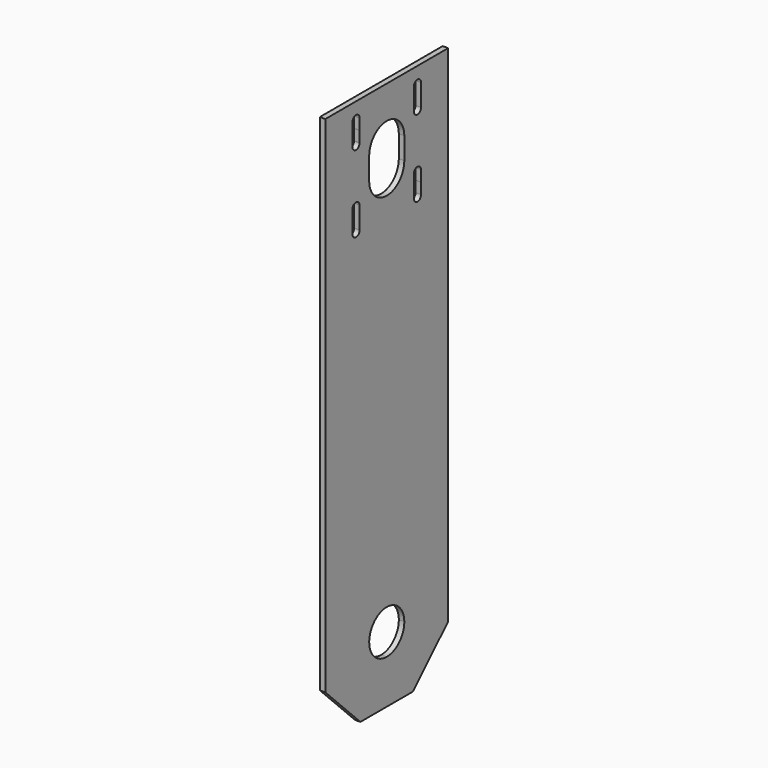
from build123d import *

# Parameters (mm, degrees)
F1_DEPTH = 6.35


# Not quite as in the source:
# - ends of sketch curves that miss each other by under 0.0002 mm in the source are joined


with BuildPart() as f1:
    # F0 (on Right) → F1 (new body)
    with BuildSketch(Plane.YZ):
        Polygon((0, 292.1), (-88.9, 292.1), (-88.9, -292.1), (-38.1, -342.9), (0, -342.9), (38.1, -342.9), (88.9, -292.1), (88.9, 292.1), align=None)
        with BuildLine():
            ThreePointArc((25.4220090151, -266.7011916637), (17.974738209, -284.6694835829), (0, -292.1011821284))
            ThreePointArc((0, -292.1011821284), (-17.9307201788, -248.7328997446), (25.4220090151, -266.7011916637))
        make_face(mode=Mode.SUBTRACT)
        with BuildLine():
            Line((-39.2938236907, 184.15), (-39.2938236907, 171.45))
            Line((-39.2938236907, 171.45), (-39.2938236907, 158.7656303343))
            ThreePointArc((-39.2938236907, 158.7656303343), (-39.2938059227, 158.7578151761), (-39.2938, 158.75))
            ThreePointArc((-39.2938, 158.75), (-44.3355371946, 153.59507064), (-49.6011180661, 158.5211308033))
            ThreePointArc((-49.6011180661, 158.5211308033), (-49.6062, 158.75), (-49.6011180661, 158.9788691967))
            Line((-49.6011180661, 158.9788691967), (-49.6011180661, 171.2211308033))
            ThreePointArc((-49.6011180661, 171.2211308033), (-49.6062, 171.45), (-49.6011180661, 171.6788691967))
            Line((-49.6011180661, 171.6788691967), (-49.6011180661, 183.9211308033))
            ThreePointArc((-49.6011180661, 183.9211308033), (-44.5722759242, 189.3047499492), (-39.2938236907, 184.1656303343))
            ThreePointArc((-39.2938236907, 184.1656303343), (-39.2938059227, 184.1578151761), (-39.2938236907, 184.15))
        make_face(mode=Mode.SUBTRACT)
        with BuildLine():
            ThreePointArc((-39.2963037105, 260.5106642339), (-39.2944259656, 260.4303418705), (-39.2938, 260.35))
            ThreePointArc((-39.2938, 260.35), (-39.2944259656, 260.2696581295), (-39.2963037105, 260.1893357661))
            Line((-39.2963037105, 260.1893357661), (-39.2963037105, 247.8106642339))
            ThreePointArc((-39.2963037105, 247.8106642339), (-39.2944259656, 247.7303418705), (-39.2938, 247.65))
            ThreePointArc((-39.2938, 247.65), (-39.2944259656, 247.5696581295), (-39.2963037105, 247.4893357661))
            ThreePointArc((-39.2963037105, 247.4893357661), (-44.5304520833, 242.4944276843), (-49.6061999953, 247.6502204525))
            Line((-49.6061999953, 247.6502204525), (-49.6056602081, 260.2753926376))
            ThreePointArc((-49.6056602081, 260.2753926376), (-49.6061999953, 260.3502204525), (-49.6056538096, 260.4250482209))
            Line((-49.6056538096, 260.4250482209), (-49.6051185467, 272.9444007144))
            ThreePointArc((-49.6051185467, 272.9444007144), (-44.583133659, 278.2044809505), (-39.2963037105, 273.2106642339))
            ThreePointArc((-39.2963037105, 273.2106642339), (-39.2944259656, 273.1303418705), (-39.2938, 273.05))
            ThreePointArc((-39.2938, 273.05), (-39.2944259656, 272.9696581295), (-39.2963037105, 272.8893357661))
            Line((-39.2963037105, 272.8893357661), (-39.2963037105, 260.5106642339))
        make_face(mode=Mode.SUBTRACT)
        with BuildLine():
            ThreePointArc((-25.4, 228.6), (-17.9605122421, 246.5605122421), (0, 254))
            ThreePointArc((0, 254), (17.9605122421, 246.5605122421), (25.4, 228.6))
            Line((25.4, 228.6), (25.4, 203.2))
            ThreePointArc((25.4, 203.2), (0, 177.8), (-25.4, 203.2))
            Line((-25.4, 203.2), (-25.4, 228.6))
        make_face(mode=Mode.SUBTRACT)
        with BuildLine():
            ThreePointArc((49.6059938769, 171.496104026), (49.606148469, 171.4730522434), (49.6062, 171.45))
            ThreePointArc((49.6062, 171.45), (49.606148469, 171.4269477566), (49.6059938769, 171.403895974))
            Line((49.6059938769, 171.403895974), (49.6059938769, 158.796104026))
            ThreePointArc((49.6059938769, 158.796104026), (49.606148469, 158.7730522434), (49.6062, 158.75))
            ThreePointArc((49.6062, 158.75), (44.4268978801, 153.5938517543), (39.294007016, 158.7962037759))
            Line((39.294007016, 158.7962037759), (39.294007016, 171.4037962241))
            ThreePointArc((39.294007016, 171.4037962241), (39.2938, 171.45), (39.294007016, 171.4962037759))
            Line((39.294007016, 171.4962037759), (39.294007016, 184.1037962241))
            ThreePointArc((39.294007016, 184.1037962241), (44.403846099, 189.3059934307), (49.6059938769, 184.196104026))
            ThreePointArc((49.6059938769, 184.196104026), (49.606148469, 184.1730522434), (49.6062, 184.15))
            ThreePointArc((49.6062, 184.15), (49.606148469, 184.1269477566), (49.6059938769, 184.103895974))
            Line((49.6059938769, 184.103895974), (49.6059938769, 171.496104026))
        make_face(mode=Mode.SUBTRACT)
        with BuildLine():
            ThreePointArc((39.2938, 273.05), (44.45, 278.2062), (49.6062, 273.05))
            Line((49.6062, 273.05), (49.6062, 260.35))
            Line((49.6062, 260.35), (49.6062, 247.65))
            ThreePointArc((49.6062, 247.65), (44.45, 242.4938), (39.2938, 247.65))
            Line((39.2938, 247.65), (39.2938, 260.35))
            Line((39.2938, 260.35), (39.2938, 273.05))
        make_face(mode=Mode.SUBTRACT)
    extrude(amount=F1_DEPTH)


solid = f1.part
